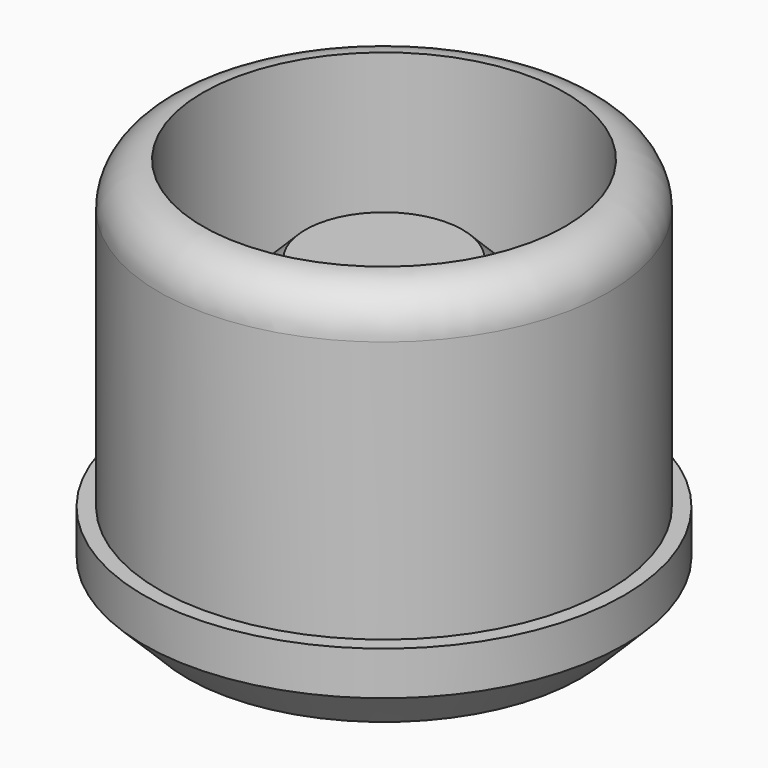
from build123d import *

# Parameters (mm, degrees)
F0_R     = 5.5
F1_DEPTH = 2
F2_R     = 2.8
F3_DEPTH = 5
F2_R_2   = 5.15
F2_R_3   = 4.15
F4_DEPTH = 7
F5_SIZE2 = 1
F5_SIZE  = 1
F6_R     = 0.99999
F7_SIZE  = 1


# Not quite as in the source:
# - a fillet or chamfer is up to 0.001 mm smaller than in the source, because OpenCascade refuses the exact size


with BuildPart() as f1:
    # F0 (on Top) → F1 (new body)
    with BuildSketch(Plane.XY):
        Circle(F0_R)
    extrude(amount=F1_DEPTH)

    # F2 (on face) → F3 (join)
    with BuildSketch(Plane.XY.offset(2)):
        Circle(F2_R)
    extrude(amount=F3_DEPTH)

    # F2 (on face) → F4 (join)
    with BuildSketch(Plane.XY.offset(2)):
        Circle(F2_R_2)
        Circle(F2_R_3, mode=Mode.SUBTRACT)
    extrude(amount=F4_DEPTH)

    # F5
    f5_edges = [f1.edges().sort_by_distance(p)[0] for p in [
        (-2.8, 0, 7),
    ]]
    chamfer(f5_edges, length=F5_SIZE, length2=F5_SIZE2)

    # F6 (radius 1 in the source; OpenCascade refuses exactly that, so slightly less here)
    f6_edges = [f1.edges().sort_by_distance(p)[0] for p in [
        (-5.15, 0, 9),
    ]]
    fillet(f6_edges, radius=F6_R)

    # F7
    f7_edges = [f1.edges().sort_by_distance(p)[0] for p in [
        (-5.5, 0, 0),
    ]]
    chamfer(f7_edges, length=F7_SIZE)


solid = f1.part
